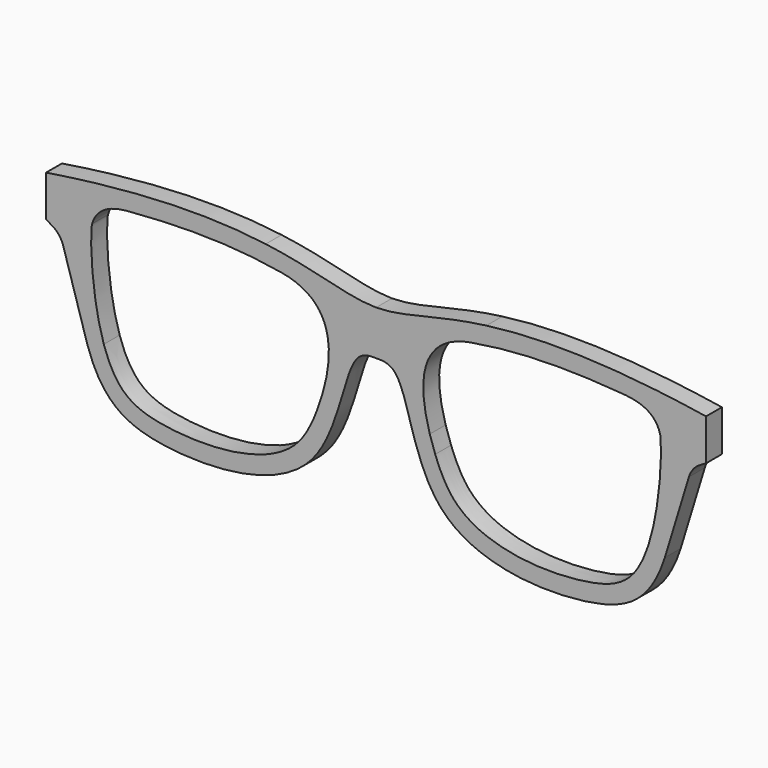
from build123d import *

# Parameters (mm, degrees)
F1_DEPTH = 4


# Not quite as in the source:
# - ends of sketch curves that miss each other by under 0.0002 mm in the source are joined
# - the dataset's text gives a spline's control points without its knots; the knots are read off the source's solid


with BuildPart() as f1:
    # F0 (on Front) → F1 (new body)
    with BuildSketch(Plane.XZ):
        with BuildLine():
            add(Edge.make_bspline(
                [(-1.43e-08, 1e-10), (-5.8262018138, 0.0296473946), (-11.5838900798, 2.612809362), (-22.2418875805, 4.0295433421)],
                knots=[0.5020838395, 0.5020838395, 0.5020838395, 0.5020838395, 0.7642308089, 0.7642308089, 0.7642308089, 0.7642308089], degree=3))
            add(Edge.make_bspline(
                [(-22.2418875765, 4.02954334), (-11.651072785, 2.4644040002), (-5.7916843406, -0.0294717417), (-1.43e-08, -1e-10)],
                knots=[0.2414899659, 0.2414899659, 0.2414899659, 0.2414899659, 0.5020838395, 0.5020838395, 0.5020838395, 0.5020838395], degree=3))
        make_face()
        with BuildLine():
            add(Edge.make_bspline(
                [(-22.2418875765, 4.02954334), (-11.651072785, 2.4644040002), (-5.7916843406, -0.0294717417), (-1.43e-08, -1e-10)],
                knots=[0.2414899659, 0.2414899659, 0.2414899659, 0.2414899659, 0.5020838395, 0.5020838395, 0.5020838395, 0.5020838395], degree=3))
            add(Edge.make_bspline(
                [(-22.2418875765, 4.02954334), (-31.827454998, 5.3037225738), (-45.3767875341, 5.6344008281), (-66.5046507984, 2.3153595296)],
                knots=[0.7642308089, 0.7642308089, 0.7642308089, 0.7642308089, 1, 1, 1, 1], degree=3))
            Line((-66.5046507984, 2.3153595296), (-66.5046507984, -6.0144829642))
            Line((-66.5046507984, -6.0144829642), (-65.3638279858, -6.6633031854))
            ThreePointArc((-65.3638279858, -6.6633031854), (-63.9321737821, -7.8850350212), (-63.0536087618, -9.5494826602))
            Line((-63.0536087618, -9.5494826602), (-58.1988021054, -25.4499952459))
            add(Edge.make_bspline(
                [(-58.1988021054, -25.4499952459), (-55.1991816547, -34.6702252334), (-44.0782715853, -40.4453435252), (-7.957963564, -38.0127679481), (-6.3941774716, -8.4142274022), (-0.7639763252, -9), (0, -9)],
                knots=[0, 0, 0, 0, 0.2689281161, 0.596888043, 0.884559193, 1, 1, 1, 1], degree=3))
            add(Edge.make_bspline(
                [(58.1988021054, -25.4499952459), (55.1991816547, -34.6702252334), (44.0782715853, -40.4453435252), (7.957963564, -38.0127679481), (6.3941774716, -8.4142274022), (0.7639763252, -9), (0, -9)],
                knots=[0, 0, 0, 0, 0.2689281161, 0.596888043, 0.884559193, 1, 1, 1, 1], degree=3))
            Line((58.1988021054, -25.4499952459), (63.0536087618, -9.5494826602))
            ThreePointArc((63.0536087618, -9.5494826602), (63.9321737821, -7.8850350212), (65.3638279858, -6.6633031854))
            Line((65.3638279858, -6.6633031854), (66.5046507984, -6.0144829642))
            Line((66.5046507984, -6.0144829642), (66.5046507984, 2.3153595296))
            add(Edge.make_bspline(
                [(22.2418875765, 4.02954334), (31.827454998, 5.3037225738), (45.3767875341, 5.6344008281), (66.5046507984, 2.3153595296)],
                knots=[0.7642308089, 0.7642308089, 0.7642308089, 0.7642308089, 1, 1, 1, 1], degree=3))
            add(Edge.make_bspline(
                [(22.2418875765, 4.02954334), (11.651072785, 2.4644040002), (5.7916843261, -0.0294717479), (-1.43e-08, 1e-10)],
                knots=[0.2414899659, 0.2414899659, 0.2414899659, 0.2414899659, 0.5020838395, 0.5020838395, 0.5020838395, 0.5020838395], degree=3))
        make_face()
        with BuildLine():
            add(Edge.make_bspline(
                [(-11.9265545389, -22.1670907577), (-11.5872866729, -21.2621257789), (-11.1962812507, -20.1593212109), (-10.8291757398, -18.933248538)],
                knots=[0, 0, 0, 0, 3.6231150837, 3.6231150837, 3.6231150837, 3.6231150837], degree=3))
            add(Edge.make_bspline(
                [(-54.8705061926, -24.3671996433), (-54.5562010662, -25.3333103894), (-53.8914718378, -27.063896226), (-52.8077601753, -29.1080753626), (-51.656094325, -30.6786246118), (-50.4280570032, -31.8827250088), (-49.0688382809, -32.8307757364), (-47.4974111469, -33.5964826314), (-45.6499849097, -34.2109611227), (-43.8574847004, -34.6093123189), (-42.2683088875, -34.8698049076), (-40.5817771148, -35.096300949), (-38.3545464684, -35.3040262976), (-35.5457216974, -35.4100418068), (-31.7086076313, -35.3320398478), (-26.8965546018, -34.7742361344), (-22.4923746975, -33.5028198227), (-19.4542274718, -32.0404045665), (-17.7957940999, -30.945241443), (-16.6273594788, -29.9605503291), (-15.9638632092, -29.2985661836), (-15.4736438559, -28.7395490718), (-14.9970074694, -28.1459612443), (-14.4297847511, -27.3450540446), (-13.7932753373, -26.2964579639), (-13.0029229552, -24.7966224837), (-12.3942573657, -23.3924139645), (-11.9982208893, -22.3582632342), (-11.9265545389, -22.1670907577)],
                knots=[0, 0, 0, 0, 0.03125, 0.0625, 0.09375, 0.125, 0.15625, 0.1875, 0.21875, 0.25, 0.265625, 0.28125, 0.3125, 0.34375, 0.375, 0.4375, 0.5, 0.53125, 0.5625, 0.578125, 0.59375, 0.6015625, 0.609375, 0.625, 0.640625, 0.65625, 0.6875, 0.694539654, 0.694539654, 0.694539654, 0.694539654], degree=3))
            add(Edge.make_bspline(
                [(-54.8705061926, -24.3671996433), (-57.5287425278, -16.1963157682), (-57.7135793865, -5.0522456877), (-57.2005584836, -3.730394179)],
                knots=[0, 0, 0, 0, 20.7679292047, 20.7679292047, 20.7679292047, 20.7679292047], degree=3))
            add(Edge.make_bspline(
                [(-50.4861483498, 0.7887146304), (-54.1156288275, 0.4196645954), (-56.4708815987, -1.0449266358), (-57.2005584836, -3.730394179)],
                knots=[0.3590211224, 0.3590211224, 0.3590211224, 0.3590211224, 8.5237816125, 8.5237816125, 8.5237816125, 8.5237816125], degree=3))
            add(Edge.make_bspline(
                [(-50, 0.8310541109), (-50.164493305, 0.819052119), (-50.3265527124, 0.8049425109), (-50.4861483498, 0.7887146304)],
                knots=[0, 0, 0, 0, 0.3590211224, 0.3590211224, 0.3590211224, 0.3590211224], degree=3))
            add(Edge.make_bspline(
                [(-19.0497534433, 3.74384e-05), (-19.7026158101, 0.1134028314), (-22.629633653, 0.5909661284), (-28.5662001971, 1.2792345618), (-38.0764085436, 1.5656807502), (-45.8463540717, 1.187404519), (-50, 0.8310541109)],
                knots=[0.7313307183, 0.7313307183, 0.7313307183, 0.7313307183, 0.75, 0.8125, 0.875, 0.9332457829, 0.9332457829, 0.9332457829, 0.9332457829], degree=3))
            add(Edge.make_bspline(
                [(-10.8291757398, -18.933248538), (-8.8371262434, -12.2801273552), (-7.5488207908, -1.9973192902), (-19.0497534433, 3.74384e-05)],
                knots=[3.6231150837, 3.6231150837, 3.6231150837, 3.6231150837, 23.2834698427, 23.2834698427, 23.2834698427, 23.2834698427], degree=3))
        make_face(mode=Mode.SUBTRACT)
        with BuildLine():
            add(Edge.make_bspline(
                [(54.8705061926, -24.3671996433), (57.5287425278, -16.1963157682), (57.7135793865, -5.0522456877), (57.2005584836, -3.730394179)],
                knots=[0, 0, 0, 0, 20.7679292047, 20.7679292047, 20.7679292047, 20.7679292047], degree=3))
            add(Edge.make_bspline(
                [(54.8705061926, -24.3671996433), (54.5562010662, -25.3333103894), (53.8914718378, -27.063896226), (52.8077601753, -29.1080753626), (51.656094325, -30.6786246118), (50.4280570032, -31.8827250088), (49.0688382809, -32.8307757364), (47.4974111469, -33.5964826314), (45.6499849097, -34.2109611227), (43.8574847004, -34.6093123189), (42.2683088875, -34.8698049076), (40.5817771148, -35.096300949), (38.3545464684, -35.3040262976), (35.5457216974, -35.4100418068), (31.7086076313, -35.3320398478), (26.8965546018, -34.7742361344), (22.4923746975, -33.5028198227), (19.4542274718, -32.0404045665), (17.7957940999, -30.945241443), (16.6273594788, -29.9605503291), (15.9638632092, -29.2985661836), (15.4736438559, -28.7395490718), (14.9970074694, -28.1459612443), (14.4297847511, -27.3450540446), (13.7932753373, -26.2964579639), (13.0029229552, -24.7966224837), (12.3942573657, -23.3924139645), (11.9982208893, -22.3582632342), (11.9265559241, -22.1670902385)],
                knots=[0, 0, 0, 0, 0.03125, 0.0625, 0.09375, 0.125, 0.15625, 0.1875, 0.21875, 0.25, 0.265625, 0.28125, 0.3125, 0.34375, 0.375, 0.4375, 0.5, 0.53125, 0.5625, 0.578125, 0.59375, 0.6015625, 0.609375, 0.625, 0.640625, 0.65625, 0.6875, 0.694539654, 0.694539654, 0.694539654, 0.694539654], degree=3))
            add(Edge.make_bspline(
                [(11.9265559241, -22.1670902385), (11.5872866729, -21.2621257789), (11.1962812507, -20.1593212109), (10.8291757398, -18.933248538)],
                knots=[0, 0, 0, 0, 3.6231150837, 3.6231150837, 3.6231150837, 3.6231150837], degree=3))
            add(Edge.make_bspline(
                [(10.8291757398, -18.933248538), (8.8371262434, -12.2801273552), (7.5488207908, -1.9973192902), (19.0497599446, 0)],
                knots=[3.6231150837, 3.6231150837, 3.6231150837, 3.6231150837, 23.2834698427, 23.2834698427, 23.2834698427, 23.2834698427], degree=3))
            add(Edge.make_bspline(
                [(19.0497599446, 0), (19.7026158101, 0.1134028314), (22.629633653, 0.5909661284), (28.5662001971, 1.2792345618), (38.0764085436, 1.5656807502), (45.8463540717, 1.187404519), (50.0000000976, 0.8310552491)],
                knots=[0.7313307183, 0.7313307183, 0.7313307183, 0.7313307183, 0.75, 0.8125, 0.875, 0.9332457829, 0.9332457829, 0.9332457829, 0.9332457829], degree=3))
            add(Edge.make_bspline(
                [(50.0000000976, 0.8310552491), (50.164493305, 0.819052119), (50.3265527124, 0.8049425109), (50.4861483498, 0.7887146304)],
                knots=[0, 0, 0, 0, 0.3590211224, 0.3590211224, 0.3590211224, 0.3590211224], degree=3))
            add(Edge.make_bspline(
                [(50.4861483498, 0.7887146304), (54.1156288275, 0.4196645954), (56.4708815987, -1.0449266358), (57.2005584836, -3.730394179)],
                knots=[0.3590211224, 0.3590211224, 0.3590211224, 0.3590211224, 8.5237816125, 8.5237816125, 8.5237816125, 8.5237816125], degree=3))
        make_face(mode=Mode.SUBTRACT)
        with BuildLine():
            add(Edge.make_bspline(
                [(-1.43e-08, -1e-10), (5.8262017929, 0.0296473883), (11.5838900664, 2.612809356), (22.2418875725, 4.0295433379)],
                knots=[0.5020838395, 0.5020838395, 0.5020838395, 0.5020838395, 0.7642308089, 0.7642308089, 0.7642308089, 0.7642308089], degree=3))
            add(Edge.make_bspline(
                [(22.2418875765, 4.02954334), (11.651072785, 2.4644040002), (5.7916843261, -0.0294717479), (-1.43e-08, 1e-10)],
                knots=[0.2414899659, 0.2414899659, 0.2414899659, 0.2414899659, 0.5020838395, 0.5020838395, 0.5020838395, 0.5020838395], degree=3))
        make_face()
    extrude(amount=-F1_DEPTH)


solid = f1.part
